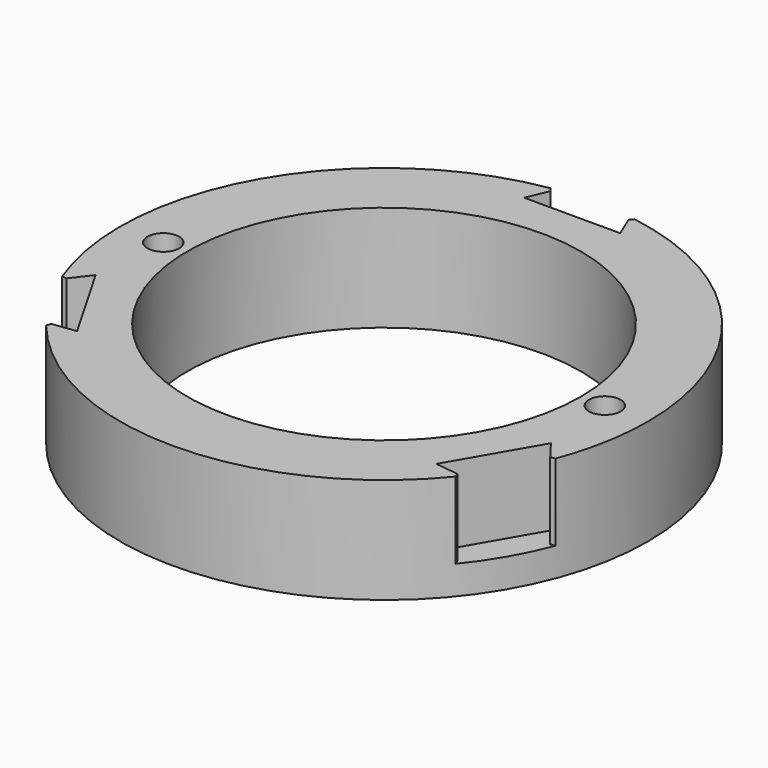
from build123d import *

# Parameters (mm, degrees)
F0_R        = 27.5
F0_R_2      = 20.5
F1_DEPTH    = 11
F2_R        = 1.65
F3_DEPTH    = 11.001
F5_DEPTH    = 8
F6_T1_DEPTH = 9.2955577349


# Not quite as in the source:
# - a fillet or chamfer that OpenCascade refuses, or shapes differently, is made with other operations: its cross-section is extruded or revolved along the edge and cut away or added


with BuildPart() as f1:
    # F0 (on Top) → F1 (new body)
    with BuildSketch(Plane.XY):
        Circle(F0_R)
        Circle(F0_R_2, mode=Mode.SUBTRACT)
    extrude(amount=F1_DEPTH)

    # F2 (on face) → F3 (cut, through all)
    with BuildSketch(Plane.XY.offset(11)):
        with Locations((-23, 0)):
            Circle(F2_R)
        with Locations((23, 0)):
            Circle(F2_R)
    extrude(amount=-F3_DEPTH, mode=Mode.SUBTRACT)

    # F4 (on face) → F5 (cut)
    with BuildSketch(Plane.XY.offset(11)):
        Polygon((2.5, 30.5), (-2.5, 30.5), (-5, 24.5), (5, 24.5), align=None)
        Polygon((-27.6637748154, -13.0849364905), (-25.1637748154, -17.4150635095), (-18.7176223927, -16.5801270189), (-23.7176223927, -7.9198729811), align=None)
        Polygon((25.1637748154, -17.4150635095), (27.6637748154, -13.0849364905), (23.7176223927, -7.9198729811), (18.7176223927, -16.5801270189), align=None)
    extrude(amount=-F5_DEPTH, mode=Mode.SUBTRACT)

    # F6: chamfer of 0.5 on 6 edges, made by hand

    # F6_s2 → F6_t1 (cut)
    with BuildSketch(Plane.XY.offset(3)):
        with BuildLine():
            Line((4.3783542155, 27.1669165233), (4.0456541802, 26.7450037593))
            Line((4.0456541802, 26.7450037593), (4.0364234109, 26.7411576055))
            ThreePointArc((4.0364234109, 26.7411576055), (3.953486728, 26.9856318529), (3.8544223971, 27.223386247))
            Line((3.8544223971, 27.223386247), (3.8650581311, 27.2371332126))
            ThreePointArc((3.8650581311, 27.2371332126), (4.1213755716, 27.1995287348), (4.3799418411, 27.1767896913))
            Line((4.3799418411, 27.1767896913), (4.3783542155, 27.1669165233))
        make_face()
        with BuildLine():
            Line((-4.3783542155, 27.1669165233), (-4.0456541802, 26.7450037593))
            Line((-4.0456541802, 26.7450037593), (-4.0364234109, 26.7411576055))
            ThreePointArc((-4.0364234109, 26.7411576055), (-3.953486728, 26.9856318529), (-3.8544223971, 27.223386247))
            Line((-3.8544223971, 27.223386247), (-3.8650581311, 27.2371332126))
            ThreePointArc((-3.8650581311, 27.2371332126), (-4.1213755716, 27.1995287348), (-4.3799418411, 27.1767896913))
            Line((-4.3799418411, 27.1767896913), (-4.3783542155, 27.1669165233))
        make_face()
        with BuildLine():
            Line((25.7164169594, -9.7916922843), (25.18467977, -9.8688625847))
            Line((25.18467977, -9.8688625847), (25.1767335184, -9.8749335884))
            ThreePointArc((25.1767335184, -9.8749335884), (25.3469860858, -10.0689959865), (25.5033552655, -10.2736654107))
            Line((25.5033552655, -10.2736654107), (25.520578354, -10.2713280777))
            ThreePointArc((25.520578354, -10.2713280777), (25.6161706411, -10.0305484239), (25.7257611865, -9.7952539442))
            Line((25.7257611865, -9.7952539442), (25.7164169594, -9.7916922843))
        make_face()
        with BuildLine():
            Line((21.3380627439, -17.3752242391), (21.1390255898, -16.8761411746))
            Line((21.1390255898, -16.8761411746), (21.1403101075, -16.866224017))
            ThreePointArc((21.1403101075, -16.866224017), (21.3934993578, -16.9166358664), (21.6489328684, -16.9497208363))
            Line((21.6489328684, -16.9497208363), (21.6555202229, -16.965805135))
            ThreePointArc((21.6555202229, -16.965805135), (21.4947950695, -17.168980311), (21.3458193454, -17.3815357471))
            Line((21.3458193454, -17.3815357471), (21.3380627439, -17.3752242391))
        make_face()
        with BuildLine():
            Line((-25.7164169594, -9.7916922843), (-25.18467977, -9.8688625847))
            Line((-25.18467977, -9.8688625847), (-25.1767335184, -9.8749335884))
            ThreePointArc((-25.1767335184, -9.8749335884), (-25.3469860858, -10.0689959865), (-25.5033552655, -10.2736654107))
            Line((-25.5033552655, -10.2736654107), (-25.520578354, -10.2713280777))
            ThreePointArc((-25.520578354, -10.2713280777), (-25.6161706411, -10.0305484239), (-25.7257611865, -9.7952539442))
            Line((-25.7257611865, -9.7952539442), (-25.7164169594, -9.7916922843))
        make_face()
        with BuildLine():
            Line((-21.3380627439, -17.3752242391), (-21.1390255898, -16.8761411746))
            Line((-21.1390255898, -16.8761411746), (-21.1403101075, -16.866224017))
            ThreePointArc((-21.1403101075, -16.866224017), (-21.3934993578, -16.9166358664), (-21.6489328684, -16.9497208363))
            Line((-21.6489328684, -16.9497208363), (-21.6555202229, -16.965805135))
            ThreePointArc((-21.6555202229, -16.965805135), (-21.4947950695, -17.168980311), (-21.3458193454, -17.3815357471))
            Line((-21.3458193454, -17.3815357471), (-21.3380627439, -17.3752242391))
        make_face()
    extrude(amount=F6_T1_DEPTH, mode=Mode.SUBTRACT)


solid = f1.part
